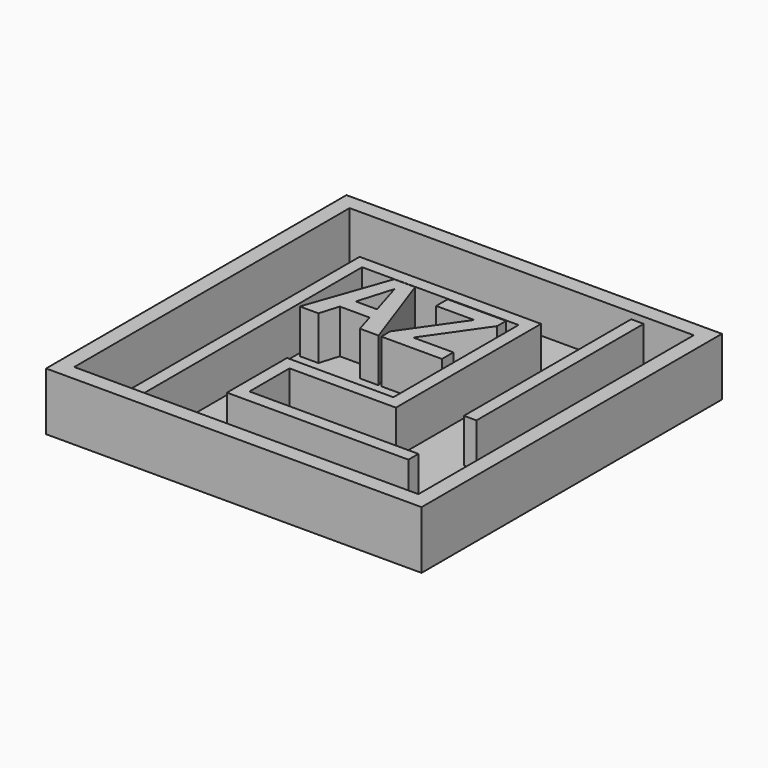
from build123d import *

# Parameters (mm, degrees)
F0_W         = 38.1
F0_H         = 38.1
F1_DEPTH     = 0.79375
F2_W         = 38.1
F2_H         = 38.1
F2_W_2       = 34.925
F2_H_2       = 34.925
F3_DEPTH     = 5.08
F4_W         = 1.27
F4_H         = 21.2153870162
F4_TEXT_SIZE = 11.5872289386
F5_DEPTH     = 4.445
F4_R         = 1.27
F6_DEPTH     = 0.396875


# Not quite as in the source:
# - Text() gives the source's letters only with a copy of the font that has no kerning and outlines rounded to 1/6400 em; it was checked with that copy


with BuildPart() as f1:
    # F0 (on Top) → F1 (new body)
    with BuildSketch(Plane.XY):
        Rectangle(F0_W, F0_H)
    extrude(amount=F1_DEPTH)

    # F2 (on face) → F3 (join)
    with BuildSketch(Plane.XY.offset(0.79375)):
        Rectangle(F2_W, F2_H)
        Rectangle(F2_W_2, F2_H_2, mode=Mode.SUBTRACT)
    extrude(amount=F3_DEPTH)

    # F4 (on face) → F5 (join)
    with BuildSketch(Plane.XY.offset(0.79375)):
        Polygon((-12.3825, 12.3825), (-12.3825, -17.4625), (-11.1125, -17.4625), (-11.1125, 11.1125), (4.7625, 11.1125), (4.7625, -4.7625), (-4.7625, -4.7625), (-6.0325, -4.7625), (-6.0325, -6.0325), (-6.0325, -12.3825), (-4.7625, -12.3825), (12.3825, -12.3825), (12.3825, -11.1125), (-4.7625, -11.1125), (-4.7625, -6.0325), (4.7625, -6.0325), (6.0325, -6.0325), (6.0325, 11.1125), (6.0325, 12.3825), (-11.1125, 12.3825), align=None)
        with Locations((11.7475, 6.8548064919)):
            Rectangle(F4_W, F4_H)
        with Locations((-10.7646349548, 2.7696951642)):
            Text('AZ', F4_TEXT_SIZE, font='Open Sans', font_style=FontStyle.BOLD, text_align=(TextAlign.LEFT, TextAlign.BOTTOM))
    extrude(amount=F5_DEPTH)

    # F4 (on face) → F6 (cut)
    with BuildSketch(Plane.XY.offset(0.79375)):
        with Locations((1.5875, -1.5875)):
            Circle(F4_R)
        with Locations((-14.9225, -14.9225)):
            Circle(F4_R)
    extrude(amount=-F6_DEPTH, mode=Mode.SUBTRACT)


solid = f1.part
